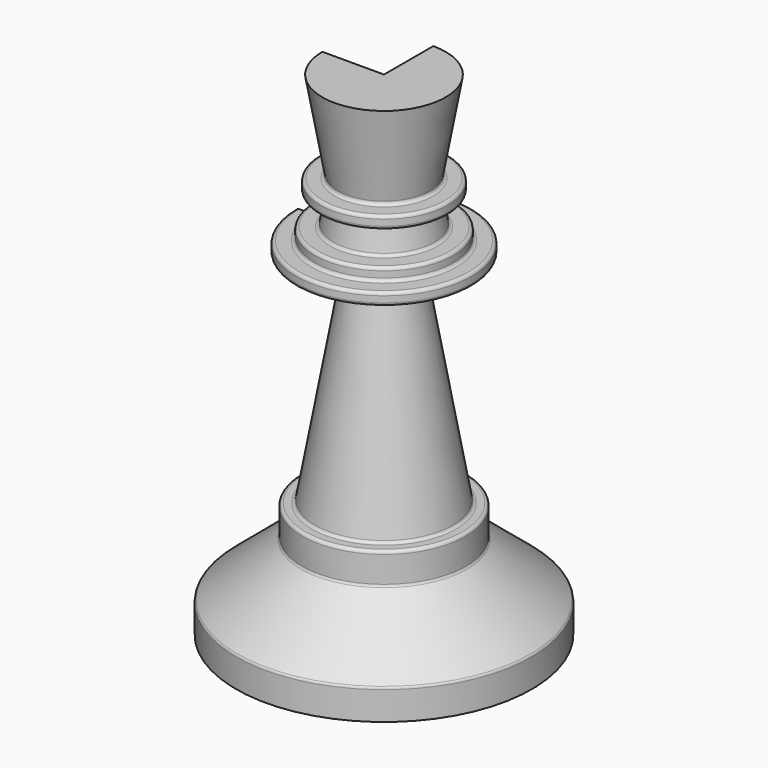
from build123d import *

# Parameters (mm, degrees)
F1_ANGLE = 270


# Not quite as in the source:
# - a feature of the source that left no trace in its solid (it failed there, or was rolled back) is left out


with BuildPart() as f1:
    # F0 (on Front) → F1 (revolve)
    with BuildSketch(Plane.XZ):
        with BuildLine():
            Line((-15.24, 0), (0, 0))
            Line((0, 0), (0, 50.8))
            Line((0, 50.8), (-6.35, 50.8))
            Line((-6.35, 50.8), (-4.7617064118, 41.792339449))
            ThreePointArc((-4.7617064118, 41.792339449), (-4.8311637627, 41.5331210865), (-5.0743828734, 41.4197061526))
            Line((-5.0743828734, 41.4197061526), (-6.2835011077, 41.4197061526))
            ThreePointArc((-6.2835011077, 41.4197061526), (-6.5080075107, 41.3267125556), (-6.6010011077, 41.1022061526))
            Line((-6.6010011077, 41.1022061526), (-6.6010011077, 40.4672061526))
            ThreePointArc((-6.6010011077, 40.4672061526), (-6.5080075107, 40.2426997495), (-6.2835011077, 40.1497061526))
            Line((-6.2835011077, 40.1497061526), (-5.0743828734, 40.1497061526))
            ThreePointArc((-5.0743828734, 40.1497061526), (-4.8311637627, 40.0362912186), (-4.7617064118, 39.7770728561))
            Line((-4.7617064118, 39.7770728561), (-5.2010717431, 37.2853082403))
            ThreePointArc((-5.2010717431, 37.2853082403), (-5.3096631386, 37.0972224261), (-5.5137482047, 37.0229415367))
            Line((-5.5137482047, 37.0229415367), (-6.8348340718, 37.0229415367))
            ThreePointArc((-6.8348340718, 37.0229415367), (-7.0593404748, 36.9299479398), (-7.1523340718, 36.7054415367))
            Line((-7.1523340718, 36.7054415367), (-7.1523340718, 36.0704415367))
            ThreePointArc((-7.1523340718, 36.0704415367), (-7.2453276688, 35.8459351337), (-7.4698340718, 35.7529415367))
            Line((-7.4698340718, 35.7529415367), (-8.7398340718, 35.7529415367))
            ThreePointArc((-8.7398340718, 35.7529415367), (-8.9643404748, 35.6599479398), (-9.0573340718, 35.4354415367))
            Line((-9.0573340718, 35.4354415367), (-9.0573340718, 34.8004415367))
            ThreePointArc((-9.0573340718, 34.8004415367), (-8.9643404748, 34.5759351337), (-8.7398340718, 34.4829415367))
            Line((-8.7398340718, 34.4829415367), (-3.5686493249, 34.4829415367))
            ThreePointArc((-3.5686493249, 34.4829415367), (-3.3254302142, 34.3695266028), (-3.2559728633, 34.1103082403))
            Line((-3.2559728633, 34.1103082403), (-7.113602572, 12.2326030065))
            ThreePointArc((-7.113602572, 12.2326030065), (-7.2221939675, 12.0445171922), (-7.4262790336, 11.9702363029))
            Line((-7.4262790336, 11.9702363029), (-8.1123649007, 11.9702363029))
            ThreePointArc((-8.1123649007, 11.9702363029), (-8.3368713037, 11.8772427059), (-8.4298649007, 11.6527363029))
            Line((-8.4298649007, 11.6527363029), (-8.4298649007, 8.9432889844))
            ThreePointArc((-8.4298649007, 8.9432889844), (-8.4596121783, 8.8091076862), (-8.5432798346, 8.7000698737))
            Line((-8.5432798346, 8.7000698737), (-15.1265850661, 3.176020882))
            ThreePointArc((-15.1265850661, 3.176020882), (-15.2102527224, 3.0669830694), (-15.24, 2.9328017713))
            Line((-15.24, 2.9328017713), (-15.24, 0))
        make_face()
    revolve(axis=Axis((0, 0, 25.4), (0, 0, 1)), revolution_arc=F1_ANGLE)


solid = f1.part
